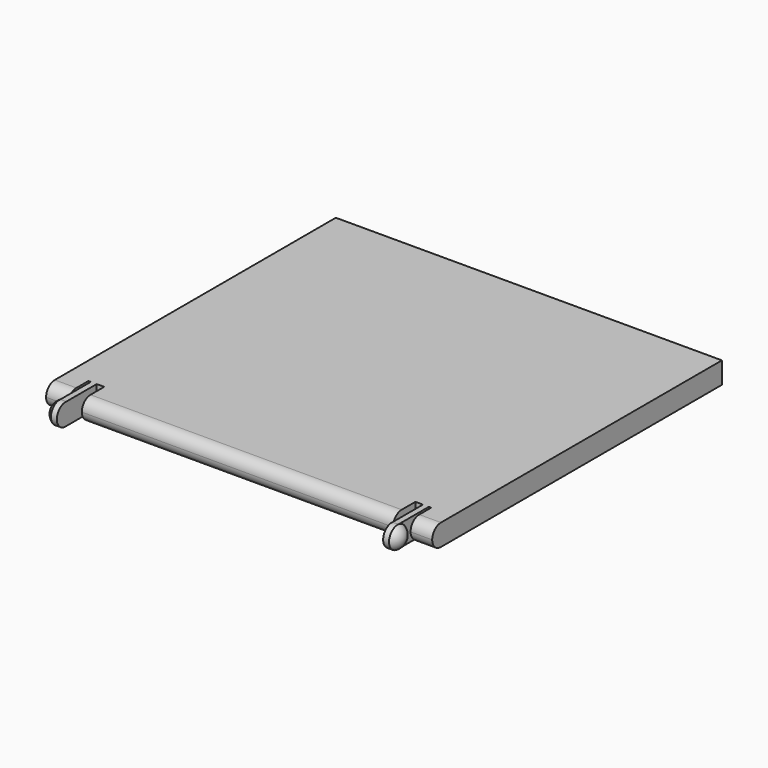
from build123d import *

# Parameters (mm, degrees)
F0_W        = 0.6898511201
F0_H        = 1.2626703829
F0_H_2      = 3.2899174839
F2_DEPTH    = 1.2573
F3_DEPTH    = 2.54
F4_T1_DEPTH = 36.3235808909
F4_T3_DEPTH = 2.5253407657
F4_T5_DEPTH = 2.5253407657


# Not quite as in the source:
# - a fillet or chamfer that OpenCascade refuses, or shapes differently, is made with other operations: its cross-section is extruded or revolved along the edge and cut away or added
# - a feature names something its author has since deleted; it is built from what else it names


with BuildPart() as f1:
    # F0 (on Top) → F1 (revolve)
    with BuildSketch(Plane.XY):
        with BuildLine():
            Line((-19.7332594544, -5.8078670874), (-19.7332594544, -4.5451967046))
            Line((-19.7332594544, -4.5451967046), (-20.5092396879, -4.5451967046))
            ThreePointArc((-20.5092396879, -4.5451967046), (-20.2997388093, -5.2862233267), (-19.7332594544, -5.8078670874))
        make_face()
        with Locations((-19.3883338943, -5.176531896)):
            Rectangle(F0_W, F0_H)
    revolve(axis=Axis((-19.3883338943, -4.5451967046, 0), (1, 0, 0)))



with BuildPart() as f1b:
    # F0 (on Top) → F1, piece 2 (revolve)
    with BuildSketch(Plane.XY):
        with BuildLine():
            Line((20.5092396879, -4.5451967046), (19.7332594544, -4.5451967046))
            Line((19.7332594544, -4.5451967046), (19.7332594544, -5.8078670874))
            ThreePointArc((19.7332594544, -5.8078670874), (20.2997388093, -5.2862233267), (20.5092396879, -4.5451967046))
        make_face()
        with Locations((19.3883338943, -5.176531896)):
            Rectangle(F0_W, F0_H)
    revolve(axis=Axis((-19.3883338943, -4.5451967046, 0), (1, 0, 0)))


with BuildPart() as f1_1:
    add(f1.part)

    add(f1b.part)  # F2 merges F1b
    # F0 (on Top) → F2 (join, symmetric)
    with BuildSketch(Plane.XY):
        Polygon((-20.009059459, 0.0073911622), (-19.7332594544, 0.0073911622), (-19.0434083343, 0.0073911622), (-18.1617904454, 0.0073911622), (-18.1617904454, -5.8078670874), (0, -5.8078670874), (18.1617904454, -5.8078670874), (18.1617904454, 0.0073911622), (19.0434083343, 0.0073911622), (19.7332594544, 0.0073911622), (20.009059459, 0.0073911622), (20.009059459, -3.01362928), (22.5344002247, -3.01362928), (22.5344002247, 39.2609333619), (0, 39.2609333619), (-22.5344002247, 39.2609333619), (-22.5344002247, -3.01362928), (-20.009059459, -3.01362928), align=None)
        with Locations((-19.3883338943, -1.6375675797)):
            Rectangle(F0_W, F0_H_2)
        with Locations((19.3883338943, -1.6375675797)):
            Rectangle(F0_W, F0_H_2)
        with Locations((-19.3883338943, -3.9138615131)):
            Rectangle(F0_W, F0_H)
        with Locations((19.3883338943, -3.9138615131)):
            Rectangle(F0_W, F0_H)
    extrude(amount=F2_DEPTH, both=True)

    # F3 (cut): a face of the model
    f3_faces = [f1_1.faces().sort_by_distance(p)[0] for p in [
        (0, -5.8078670874, 0),
    ]]
    extrude(f3_faces, amount=-F3_DEPTH, mode=Mode.SUBTRACT)

    # F4: fillet of radius 1.27 on 6 edges, made by hand

    # F4_s2 → F4_t1 (cut)
    with BuildSketch(Plane.YZ.offset(-18.1617904454)):
        with BuildLine():
            ThreePointArc((-1.9978670874, 1.2573), (-2.8958926995, 0.8853256121), (-3.2678670874, -0.0127))
            Line((-3.2678670874, -0.0127), (-3.2932670874, -0.0127))
            Line((-3.2932670874, -0.0127), (-3.2932670874, 1.2827))
            Line((-3.2932670874, 1.2827), (-1.9978670874, 1.2827))
            Line((-1.9978670874, 1.2827), (-1.9978670874, 1.2573))
        make_face()
        with BuildLine():
            ThreePointArc((-1.9978670874, -1.2573), (-2.8958926995, -0.8853256121), (-3.2678670874, 0.0127))
            Line((-3.2678670874, 0.0127), (-3.2932670874, 0.0127))
            Line((-3.2932670874, 0.0127), (-3.2932670874, -1.2827))
            Line((-3.2932670874, -1.2827), (-1.9978670874, -1.2827))
            Line((-1.9978670874, -1.2827), (-1.9978670874, -1.2573))
        make_face()
    extrude(amount=F4_T1_DEPTH, mode=Mode.SUBTRACT)

    # F4_s4 → F4_t3 (cut)
    with BuildSketch(Plane.YZ.offset(-22.5344002247)):
        with BuildLine():
            ThreePointArc((-1.74362928, 1.2573), (-2.6416548921, 0.8853256121), (-3.01362928, -0.0127))
            Line((-3.01362928, -0.0127), (-3.03902928, -0.0127))
            Line((-3.03902928, -0.0127), (-3.03902928, 1.2827))
            Line((-3.03902928, 1.2827), (-1.74362928, 1.2827))
            Line((-1.74362928, 1.2827), (-1.74362928, 1.2573))
        make_face()
        with BuildLine():
            ThreePointArc((-1.74362928, -1.2573), (-2.6416548921, -0.8853256121), (-3.01362928, 0.0127))
            Line((-3.01362928, 0.0127), (-3.03902928, 0.0127))
            Line((-3.03902928, 0.0127), (-3.03902928, -1.2827))
            Line((-3.03902928, -1.2827), (-1.74362928, -1.2827))
            Line((-1.74362928, -1.2827), (-1.74362928, -1.2573))
        make_face()
    extrude(amount=F4_T3_DEPTH, mode=Mode.SUBTRACT)

    # F4_s6 → F4_t5 (cut)
    with BuildSketch(Plane.YZ.offset(20.009059459)):
        with BuildLine():
            ThreePointArc((-1.74362928, 1.2573), (-2.6416548921, 0.8853256121), (-3.01362928, -0.0127))
            Line((-3.01362928, -0.0127), (-3.03902928, -0.0127))
            Line((-3.03902928, -0.0127), (-3.03902928, 1.2827))
            Line((-3.03902928, 1.2827), (-1.74362928, 1.2827))
            Line((-1.74362928, 1.2827), (-1.74362928, 1.2573))
        make_face()
        with BuildLine():
            ThreePointArc((-1.74362928, -1.2573), (-2.6416548921, -0.8853256121), (-3.01362928, 0.0127))
            Line((-3.01362928, 0.0127), (-3.03902928, 0.0127))
            Line((-3.03902928, 0.0127), (-3.03902928, -1.2827))
            Line((-3.03902928, -1.2827), (-1.74362928, -1.2827))
            Line((-1.74362928, -1.2827), (-1.74362928, -1.2573))
        make_face()
    extrude(amount=F4_T5_DEPTH, mode=Mode.SUBTRACT)


solid = f1_1.part
